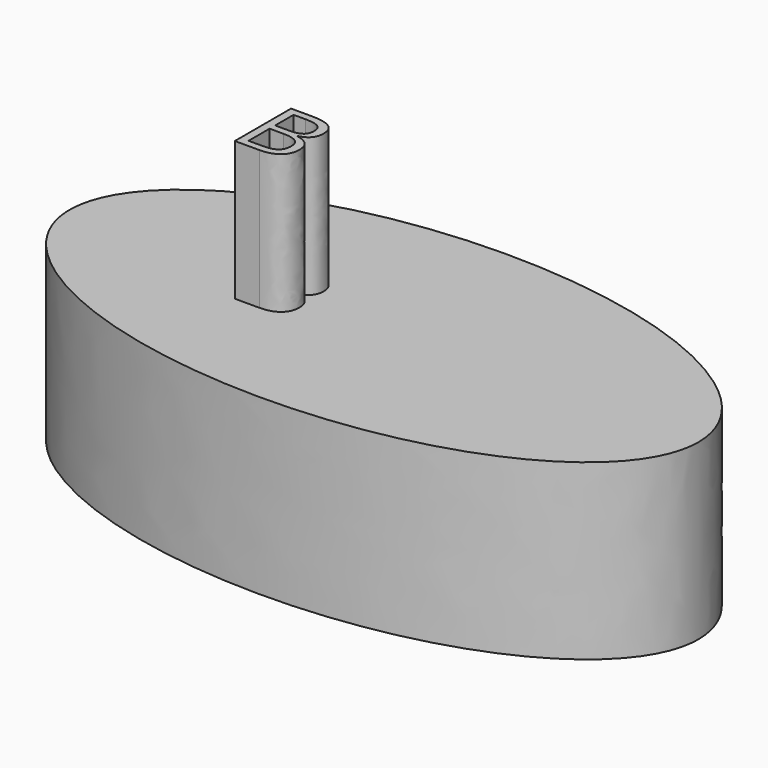
from build123d import *

# Parameters (mm, degrees)
F1_DEPTH     = 34.29
F2_TEXT_SIZE = 19.4453504971
F3_DEPTH     = 27.432


# Not quite as in the source:
# - Text() gives the source's letters only with a copy of the font that has no kerning and outlines rounded to 1/6400 em; it was checked with that copy


with BuildPart() as f1:
    # F0 (on Top) → F1 (new body)
    with BuildSketch(Plane.XY):
        with BuildLine():
            add(Edge.make_bspline(
                [(62.1219053864, 0), (62.1219053864, 52.9098048061), (-31.0609526932, 26.454902403), (-124.2438107729, 0), (-31.0609526932, -26.454902403), (62.1219053864, -52.9098048061), (62.1219053864, 0)],
                knots=[0, 0, 0, 2.0943951024, 2.0943951024, 4.1887902048, 4.1887902048, 6.2831853072, 6.2831853072, 6.2831853072], degree=2, weights=[1, 0.5, 1, 0.5, 1, 0.5, 1]))
        make_face()
    extrude(amount=F1_DEPTH)

    # F2 (on face) → F3 (join)
    with BuildSketch(Plane.XY.offset(34.29)):
        with Locations((-25.5633499473, -7.2662122548)):
            Text('B', F2_TEXT_SIZE, font='Open Sans', text_align=(TextAlign.LEFT, TextAlign.BOTTOM))
    extrude(amount=F3_DEPTH)


solid = f1.part
